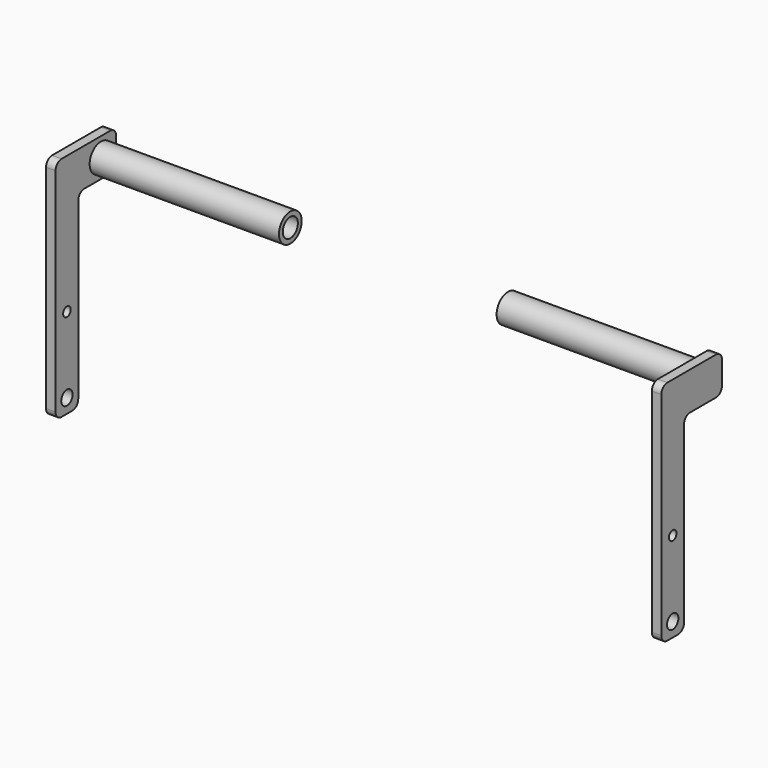
from build123d import *

# Parameters (mm, degrees)
F0_W     = 31.75
F0_H     = 25.4
F1_DEPTH = 6.35
F2_R     = 9.525
F2_R_2   = 6.35
F3_DEPTH = 127
F4_R     = 5
F5_R     = 4.7625
F5_R_2   = 3.175
F6_DEPTH = 6.351


# Not quite as in the source:
# - a length typed as a fraction of an inch, garbled in the dataset ("3 / 203.2 mm" for 3/8 in), is restored


with BuildPart() as f1:
    # F0 (on Right) → F1 (new body)
    with BuildSketch(Plane.YZ):
        Polygon((-9.525, 152.4), (-9.525, 0), (9.525, 0), (9.525, 127), (9.525, 152.4), align=None)
        with Locations((25.4, 139.7)):
            Rectangle(F0_W, F0_H)
    extrude(amount=-F1_DEPTH)

    # F2 (on face) → F3 (join)
    with BuildSketch(Plane.YZ):
        with Locations((28.575, 139.7)):
            Circle(F2_R)
        with Locations((28.575, 139.7)):
            Circle(F2_R_2, mode=Mode.SUBTRACT)
    extrude(amount=F3_DEPTH)

    # F4
    f4_edges = [f1.edges().sort_by_distance(p)[0] for p in [
        (-3.175, -9.525, 152.4),
        (-3.175, 9.525, 127),
        (-3.175, 41.275, 127),
        (-3.175, 41.275, 152.4),
        (-3.175, 9.525, 0),
        (-3.175, -9.525, 0),
    ]]
    fillet(f4_edges, radius=F4_R)

    # F5 (on face) → F6 (cut, through all)
    with BuildSketch(Plane.YZ):
        with Locations((0, 9.525)):
            Circle(F5_R)
        with Locations((0, 60.325)):
            Circle(F5_R_2)
    extrude(amount=-F6_DEPTH, mode=Mode.SUBTRACT)


with BuildPart() as f8_1:
    # F8: instance of F1
    add(f1.part.mirror(Plane.YZ.offset(200)))


solid = Compound([f1.part, f8_1.part])
